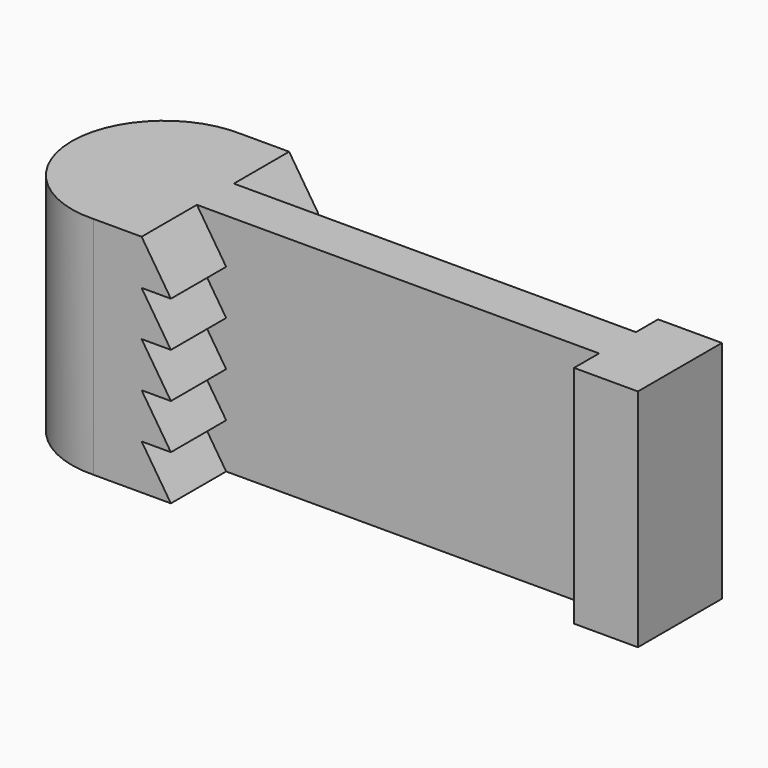
from build123d import *

# Parameters (mm, degrees)
F0_W     = 1.9128494449
F0_H     = 2
F1_DEPTH = 9.779
F3_DEPTH = 3
F5_DEPTH = 3


# Not quite as in the source:
# - a feature names something its author has since deleted; it is built from what else it names


with BuildPart() as f1:
    # F0 (on Top) → F1 (new body)
    with BuildSketch(Plane.XY):
        Polygon((14.9611846233, 0.28775621), (14.9611846233, -0.9137945543), (14.9611846233, -2.9137945543), (14.9611846233, -4.2726983058), (17.7320937316, -4.2726983058), (17.7320937316, 0.28775621), align=None)
        with BuildLine():
            Line((13.0483351785, -0.9137945543), (-0.8558859308, -0.9137945543))
            ThreePointArc((-0.8558859308, -0.9137945543), (-0.7608167592, -1.4097829714), (-0.7289579861, -1.9137945543))
            ThreePointArc((-0.7289579861, -1.9137945543), (-0.7608167592, -2.4178061373), (-0.8558859308, -2.9137945543))
            Line((-0.8558859308, -2.9137945543), (13.0483351785, -2.9137945543))
            Line((13.0483351785, -2.9137945543), (13.0483351785, -0.9137945543))
        make_face()
        with Locations((14.0047599009, -1.9137945543)):
            Rectangle(F0_W, F0_H)
        with BuildLine():
            Line((-4.7316648215, -2.9137945543), (-4.7316648215, -0.9137945543))
            Line((-4.7316648215, -0.9137945543), (-4.7316648215, 2.0862054457))
            Line((-4.7316648215, 2.0862054457), (-4.5844846254, 2.0862054457))
            ThreePointArc((-4.5844846254, 2.0862054457), (-8.7343716569, -1.9137945543), (-4.5844846254, -5.9137945543))
            Line((-4.5844846254, -5.9137945543), (-4.7316648215, -5.9137945543))
            Line((-4.7316648215, -5.9137945543), (-4.7316648215, -2.9137945543))
        make_face()
        with BuildLine():
            Line((-1.2312275376, -2.9137945543), (-4.7316648215, -2.9137945543))
            Line((-4.7316648215, -2.9137945543), (-4.7316648215, -5.9137945543))
            Line((-4.7316648215, -5.9137945543), (-4.5844846254, -5.9137945543))
            ThreePointArc((-4.5844846254, -5.9137945543), (-2.6374223247, -5.3249249204), (-1.2312275376, -3.8550830006))
            Line((-1.2312275376, -3.8550830006), (-1.2312275376, -2.9137945543))
        make_face()
        with BuildLine():
            Line((-4.7316648215, 2.0862054457), (-4.7316648215, -0.9137945543))
            Line((-4.7316648215, -0.9137945543), (-1.2264648215, -0.9137945543))
            Line((-1.2264648215, -0.9137945543), (-1.2264648215, 0.0188810444))
            ThreePointArc((-1.2264648215, 0.0188810444), (-2.6332302099, 1.4947585391), (-4.5844846254, 2.0862054457))
            Line((-4.5844846254, 2.0862054457), (-4.7316648215, 2.0862054457))
        make_face()
        with BuildLine():
            Line((-1.2264648215, -0.9137945543), (-4.7316648215, -0.9137945543))
            Line((-4.7316648215, -0.9137945543), (-4.7316648215, -2.9137945543))
            Line((-4.7316648215, -2.9137945543), (-1.2312275376, -2.9137945543))
            Line((-1.2312275376, -2.9137945543), (-0.8558859308, -2.9137945543))
            ThreePointArc((-0.8558859308, -2.9137945543), (-0.7608167592, -2.4178061373), (-0.7289579861, -1.9137945543))
            ThreePointArc((-0.7289579861, -1.9137945543), (-0.7608167592, -1.4097829714), (-0.8558859308, -0.9137945543))
            Line((-0.8558859308, -0.9137945543), (-1.2264648215, -0.9137945543))
        make_face()
        with BuildLine():
            Line((-1.2312275376, -5.9137945543), (-1.2312275376, -3.8550830006))
            ThreePointArc((-1.2312275376, -3.8550830006), (-2.6374223247, -5.3249249204), (-4.5844846254, -5.9137945543))
            Line((-4.5844846254, -5.9137945543), (-1.2312275376, -5.9137945543))
        make_face()
        with BuildLine():
            ThreePointArc((-4.5844846254, 2.0862054457), (-2.6332302099, 1.4947585391), (-1.2264648215, 0.0188810444))
            Line((-1.2264648215, 0.0188810444), (-1.2264648215, 2.0862054457))
            Line((-1.2264648215, 2.0862054457), (-4.5844846254, 2.0862054457))
        make_face()
    extrude(amount=F1_DEPTH)

    # F2 (on face) → F3 (cut)
    with BuildSketch(Plane.XZ.offset(5.9137945543)):
        Polygon((-1.2312275376, 0), (-1.2312275376, 1.9558), (-2.5021124942, 1.9558), align=None)
        Polygon((-1.2312275376, 1.9558), (-1.2312275376, 3.9116), (-2.5021124942, 3.9116), align=None)
        Polygon((-1.2312275376, 4.8895), (-1.2312275376, 5.8674), (-2.5021124942, 5.8674), (-1.2312275376, 3.9116), align=None)
        Polygon((-1.2312275376, 5.8674), (-1.2312275376, 7.8232), (-2.5021124942, 7.8232), align=None)
        Polygon((-1.2312275376, 9.779), (-2.5021124942, 9.779), (-1.2312275376, 7.8232), align=None)
    extrude(amount=-F3_DEPTH, mode=Mode.SUBTRACT)

    # F4 (on face) → F5 (cut)
    with BuildSketch(Plane(origin=(0, 2.0862054457, 0), x_dir=(-1, 0, 0), z_dir=(0, 1, 0))):
        Polygon((1.2264648215, 9.779), (1.2264648215, 7.8232), (2.4964648215, 9.779), align=None)
        Polygon((1.2264648215, 7.8232), (1.2264648215, 5.8674), (2.4964648215, 7.8232), align=None)
        Polygon((1.2264648215, 4.8895), (1.2264648215, 3.9116), (2.4964648215, 5.8674), (1.2264648215, 5.8674), align=None)
        Polygon((1.2264648215, 3.9116), (1.2264648215, 1.9558), (2.4964648215, 3.9116), align=None)
        Polygon((1.2264648215, 1.9558), (1.2264648215, 0), (2.4964648215, 1.9558), align=None)
    extrude(amount=-F5_DEPTH, mode=Mode.SUBTRACT)


solid = f1.part
